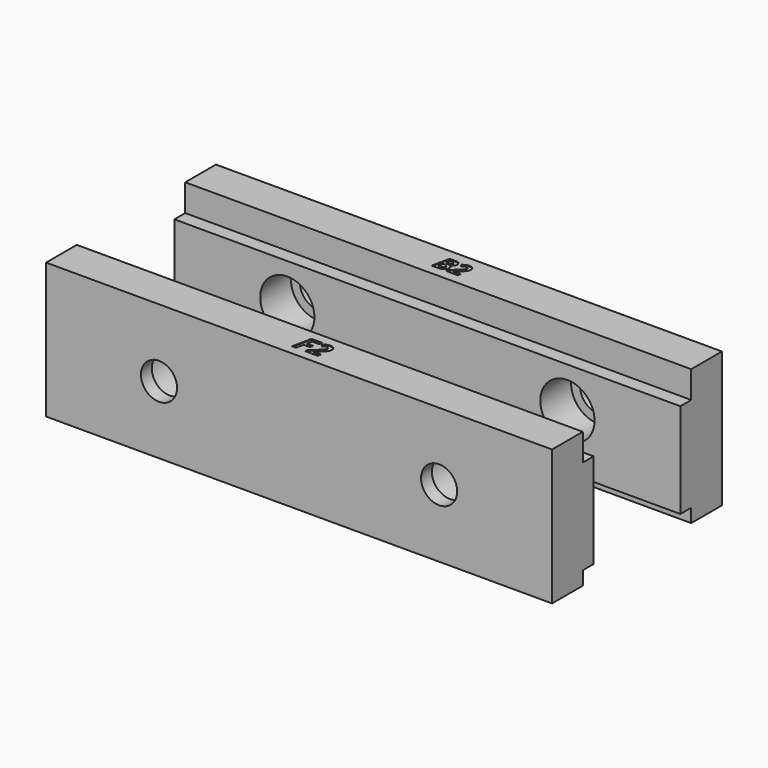
from build123d import *

# Parameters (mm, degrees)
F1_DEPTH       = 88.9
F1_DEPTH_BACK  = 88.9
F3_D           = 12.7
F3_CBORE_D     = 19.05
F3_CBORE_DEPTH = 13.49375
F5_D           = 12.7
F5_CBORE_D     = 19.05
F5_CBORE_DEPTH = 13.49375
F6_R           = 3.175
F7_DEPTH       = 9.525
F8_TEXT_SIZE   = 8.8194444444
F8_TEXT_SIZE_2 = 9.5159406784
F9_DEPTH       = 0.254


# Not quite as in the source:
# - Text() gives the source's letters only with a copy of the font that has no kerning and outlines rounded to 1/6400 em; it was checked with that copy


with BuildPart() as f1:
    # F0 (on Right) → F1 (new body, two sides)
    with BuildSketch(Plane.YZ) as f1_sk:
        Polygon((30.95625, 47.625), (17.4625, 47.625), (17.4625, 38.1), (12.7, 38.1), (12.7, 4.7625), (17.4625, 4.7625), (17.4625, 0), (30.95625, 0), align=None)
    extrude(amount=F1_DEPTH)
    extrude(f1_sk.sketch, amount=-F1_DEPTH_BACK)

    # F5 (through all)
    with Locations(Plane.XZ.offset(-12.7)):
        with Locations((-49.2125, 23.8125), (49.2125, 23.8125)):
            CounterBoreHole(F5_D / 2, F5_CBORE_D / 2, F5_CBORE_DEPTH)

    # F6 (on face) → F7 (cut)
    with BuildSketch(Plane(origin=(0, 30.95625, 0), x_dir=(-1, 0, 0), z_dir=(0, 1, 0))):
        with Locations((-79.375, 31.75)):
            Circle(F6_R)
    extrude(amount=-F7_DEPTH, mode=Mode.SUBTRACT)


with BuildPart() as f1b:
    # F0 (on Right) → F1, piece 2 (new body, two sides)
    with BuildSketch(Plane.YZ) as f1_2_sk:
        Polygon((-17.4625, 38.1), (-17.4625, 47.625), (-30.95625, 47.625), (-30.95625, 0), (-17.4625, 0), (-17.4625, 4.7625), (-12.7, 4.7625), (-12.7, 38.1), align=None)
    extrude(amount=F1_DEPTH)
    extrude(f1_2_sk.sketch, amount=-F1_DEPTH_BACK)

    # F3 (through all)
    with Locations(Plane(origin=(0, -12.7, 0), x_dir=(-1, 0, 0), z_dir=(0, 1, 0))):
        with Locations((-49.2125, 23.8125), (49.2125, 23.8125)):
            CounterBoreHole(F3_D / 2, F3_CBORE_D / 2, F3_CBORE_DEPTH)


with BuildPart() as f9_tool:
    # F8 (on face) → F9 (new body)
    with BuildSketch(Plane.XY.offset(47.625)):
        with Locations((-5.3846842448, 21.034375)):
            Text('B2', F8_TEXT_SIZE, font='Open Sans', font_style=FontStyle.BOLDITALIC, text_align=(TextAlign.LEFT, TextAlign.BOTTOM))
        with Locations((-5.3846842448, -27.6351136442)):
            Text('F2', F8_TEXT_SIZE_2, font='Open Sans', font_style=FontStyle.BOLDITALIC, text_align=(TextAlign.LEFT, TextAlign.BOTTOM))
    extrude(amount=-F9_DEPTH)


with BuildPart() as f1_1:
    add(f1.part)

    # F9: cut by f9_tool
    add(f9_tool.part, mode=Mode.SUBTRACT)


with BuildPart() as f1b_1:
    add(f1b.part)

    # F9: cut by f9_tool
    add(f9_tool.part, mode=Mode.SUBTRACT)


with BuildPart() as f1b_2:
    # F10: moved
    add(f1b_1.part.moved(Location((0, -12.7, 0))))


solid = Compound([f1_1.part, f1b_2.part])
